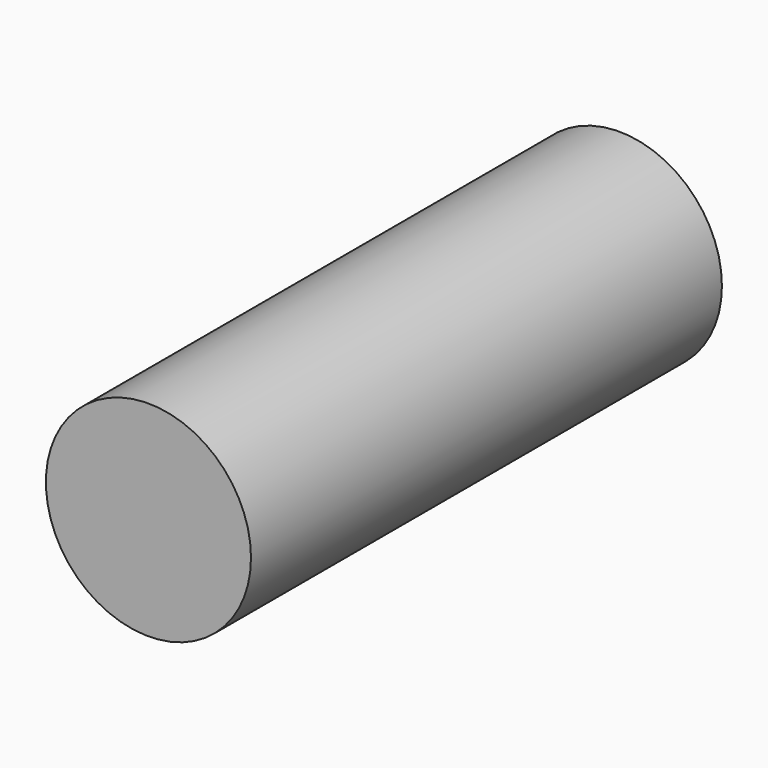
from build123d import *

# Parameters (mm, degrees)
F0_R     = 12.7
F1_DEPTH = 72.898
F4_R     = 7.62
F5_DEPTH = 127


# Not quite as in the source:
# - the program builds the solid bodies; features that only make, move or delete a surface that nothing else refers to are left out


with BuildPart() as f1:
    # F0 (on Front) → F1 (new body)
    with BuildSketch(Plane.XZ):
        Circle(F0_R)
    extrude(amount=F1_DEPTH)

    # F4 (on face) → F5 (cut)
    with BuildSketch(Plane(origin=(0, 0, 0), x_dir=(-1, 0, 0), z_dir=(0, 1, 0))):
        with Locations((0, -25.8763151404)):
            Circle(F4_R)
    extrude(amount=-F5_DEPTH, mode=Mode.SUBTRACT)


solid = f1.part
